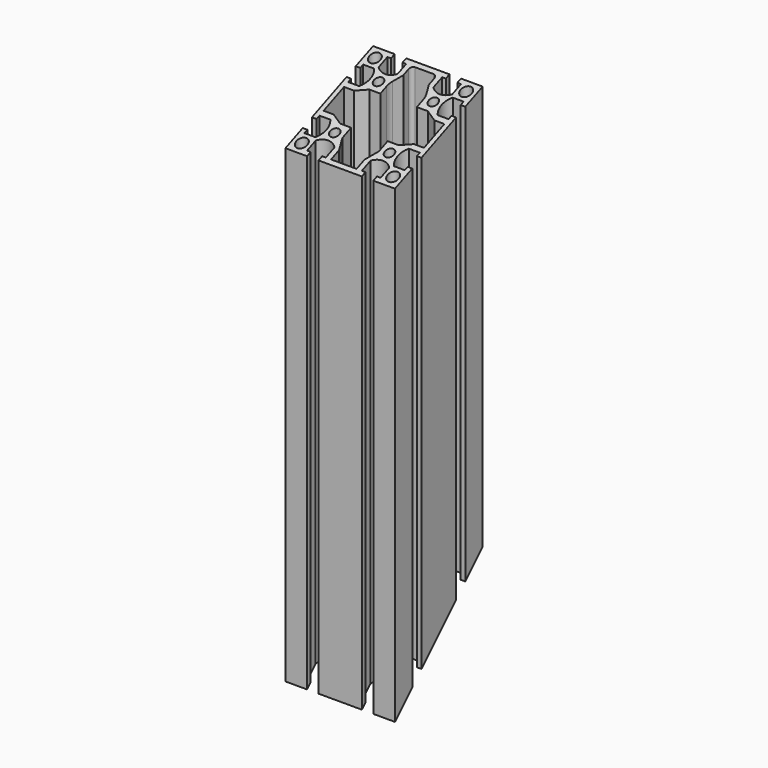
from build123d import *

# Parameters (mm, degrees)
F0_R          = 3
F0_R_2        = 2.5
F1_DEPTH      = 282
F2_R          = 2
F3_R          = 7
F6_DEPTH      = 30
F6_DEPTH_BACK = 30


# Not quite as in the source:
# - a feature names something its author has since deleted; it is built from what else it names


with BuildPart() as f1:
    # F0 (on Top) → F1 (new body)
    with BuildSketch(Plane.XY):
        with BuildLine():
            Line((18.15, -30), (30, -30))
            Line((30, -30), (30, -18.15))
            Line((30, -18.15), (27.5, -18.15))
            Line((27.5, -18.15), (27.5, -20.15))
            Line((27.5, -20.15), (21.5477069044, -20.15))
            ThreePointArc((21.5477069044, -20.15), (19.5, -15), (21.5477069044, -9.85))
            Line((21.5477069044, -9.85), (27.5, -9.85))
            Line((27.5, -9.85), (27.5, -11.85))
            Line((27.5, -11.85), (30, -11.85))
            Line((30, -11.85), (30, 11.85))
            Line((30, 11.85), (27.5, 11.85))
            Line((27.5, 11.85), (27.5, 9.85))
            Line((27.5, 9.85), (21.5477069044, 9.85))
            ThreePointArc((21.5477069044, 9.85), (19.5, 15), (21.5477069044, 20.15))
            Line((21.5477069044, 20.15), (27.5, 20.15))
            Line((27.5, 20.15), (27.5, 18.15))
            Line((27.5, 18.15), (30, 18.15))
            Line((30, 18.15), (30, 30))
            Line((30, 30), (18.15, 30))
            Line((18.15, 30), (18.15, 27.5))
            Line((18.15, 27.5), (20.15, 27.5))
            Line((20.15, 27.5), (20.15, 21.5477069044))
            ThreePointArc((20.15, 21.5477069044), (15, 19.5), (9.85, 21.5477069044))
            Line((9.85, 21.5477069044), (9.85, 27.5))
            Line((9.85, 27.5), (11.85, 27.5))
            Line((11.85, 27.5), (11.85, 30))
            Line((11.85, 30), (-11.85, 30))
            Line((-11.85, 30), (-11.85, 27.5))
            Line((-11.85, 27.5), (-9.85, 27.5))
            Line((-9.85, 27.5), (-9.85, 21.5477069044))
            ThreePointArc((-9.85, 21.5477069044), (-15, 19.5), (-20.15, 21.5477069044))
            Line((-20.15, 21.5477069044), (-20.15, 27.5))
            Line((-20.15, 27.5), (-18.15, 27.5))
            Line((-18.15, 27.5), (-18.15, 30))
            Line((-18.15, 30), (-30, 30))
            Line((-30, 30), (-30, 18.15))
            Line((-30, 18.15), (-27.5, 18.15))
            Line((-27.5, 18.15), (-27.5, 20.15))
            Line((-27.5, 20.15), (-21.5477069044, 20.15))
            ThreePointArc((-21.5477069044, 20.15), (-19.5, 15), (-21.5477069044, 9.85))
            Line((-21.5477069044, 9.85), (-27.5, 9.85))
            Line((-27.5, 9.85), (-27.5, 11.85))
            Line((-27.5, 11.85), (-30, 11.85))
            Line((-30, 11.85), (-30, -11.85))
            Line((-30, -11.85), (-27.5, -11.85))
            Line((-27.5, -11.85), (-27.5, -9.85))
            Line((-27.5, -9.85), (-21.5477069044, -9.85))
            ThreePointArc((-21.5477069044, -9.85), (-19.5, -15), (-21.5477069044, -20.15))
            Line((-21.5477069044, -20.15), (-27.5, -20.15))
            Line((-27.5, -20.15), (-27.5, -18.15))
            Line((-27.5, -18.15), (-30, -18.15))
            Line((-30, -18.15), (-30, -30))
            Line((-30, -30), (-18.15, -30))
            Line((-18.15, -30), (-18.15, -27.5))
            Line((-18.15, -27.5), (-20.15, -27.5))
            Line((-20.15, -27.5), (-20.15, -21.5477069044))
            ThreePointArc((-20.15, -21.5477069044), (-15, -19.5), (-9.85, -21.5477069044))
            Line((-9.85, -21.5477069044), (-9.85, -27.5))
            Line((-9.85, -27.5), (-11.85, -27.5))
            Line((-11.85, -27.5), (-11.85, -30))
            Line((-11.85, -30), (11.85, -30))
            Line((11.85, -30), (11.85, -27.5))
            Line((11.85, -27.5), (9.85, -27.5))
            Line((9.85, -27.5), (9.85, -21.5477069044))
            ThreePointArc((9.85, -21.5477069044), (15, -19.5), (20.15, -21.5477069044))
            Line((20.15, -21.5477069044), (20.15, -27.5))
            Line((20.15, -27.5), (18.15, -27.5))
            Line((18.15, -27.5), (18.15, -30))
        make_face()
        with Locations((-25, -25)):
            Circle(F0_R, mode=Mode.SUBTRACT)
        with Locations((-15, -15)):
            Circle(F0_R_2, mode=Mode.SUBTRACT)
        with Locations((25, -25)):
            Circle(F0_R, mode=Mode.SUBTRACT)
        with Locations((15, -15)):
            Circle(F0_R_2, mode=Mode.SUBTRACT)
        with Locations((-25, 25)):
            Circle(F0_R, mode=Mode.SUBTRACT)
        with Locations((-15, 15)):
            Circle(F0_R_2, mode=Mode.SUBTRACT)
        Polygon((-7, 22), (-7, 27.5), (0, 27.5), (7, 27.5), (7, 22), (10, 16), (10, 10), (16, 10), (22, 7), (27.5, 7), (27.5, 0), (27.5, -7), (22, -7), (16, -10), (10, -10), (10, -16), (7, -22), (7, -27.5), (0, -27.5), (-7, -27.5), (-7, -22), (-10, -16), (-10, -10), (-16, -10), (-22, -7), (-27.5, -7), (-27.5, 0), (-27.5, 7), (-22, 7), (-16, 10), (-10, 10), (-10, 16), align=None, mode=Mode.SUBTRACT)
        with Locations((15, 15)):
            Circle(F0_R_2, mode=Mode.SUBTRACT)
        with Locations((25, 25)):
            Circle(F0_R, mode=Mode.SUBTRACT)
    extrude(amount=F1_DEPTH)

    # F2
    f2_edges = [f1.edges().sort_by_distance(p)[0] for p in [
        (-7, 27.5, 141),
        (7, 27.5, 141),
    ]]
    fillet(f2_edges, radius=F2_R)

    # F3
    f3_edges = [f1.edges().sort_by_distance(p)[0] for p in [
        (-10, 16, 141),
        (10, 16, 141),
    ]]
    fillet(f3_edges, radius=F3_R)

    # F5 (on Right) → F6 (cut, two sides)
    with BuildSketch(Plane.YZ) as f6_sk:
        Polygon((115.2614038106, 44.5196963257), (64.8905500682, 94.8905500682), (-30, 0), (20.3708537424, -50.3708537424), align=None)
        Polygon((30, 282), (-7.7241411908, 373.0741332917), (-157.9632044753, 310.843075681), (-120.2390632845, 219.7689423893), align=None)
    extrude(amount=F6_DEPTH, mode=Mode.SUBTRACT)
    extrude(f6_sk.sketch, amount=-F6_DEPTH_BACK, mode=Mode.SUBTRACT)


solid = f1.part
